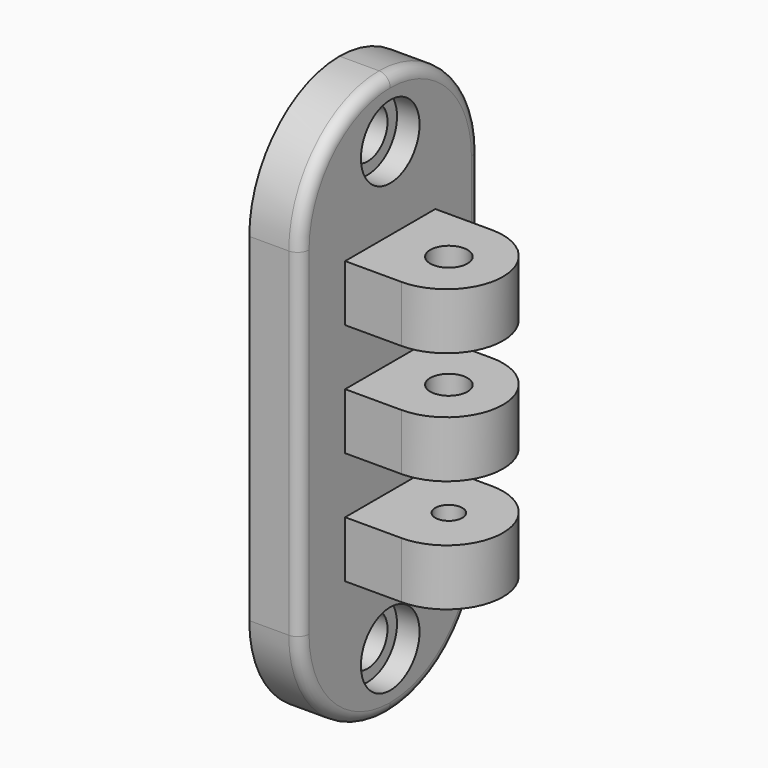
from build123d import *

# Parameters (mm, degrees)
F0_R          = 3.25
F0_W          = 10
F0_H          = 5
F0_R_2        = 2.2
F2_DEPTH      = 4.5
F3_DEPTH      = 10
F1_R          = 1.65
F1_R_2        = 1.2
F4_DEPTH      = 25
F5_DEPTH      = 2.5
F5_DEPTH_BACK = 12.5
F6_START      = -6.1
F6_DEPTH      = 8.5
F7_DEPTH      = 2
F8_R          = 1


with BuildPart() as f2:
    # F0 (on Right) → F2 (new body)
    with BuildSketch(Plane.YZ):
        with BuildLine():
            ThreePointArc((0, 25), (-7.0710678119, 22.0710678119), (-10, 15))
            Line((-10, 15), (-10, -15))
            ThreePointArc((-10, -15), (-7.0710678119, -22.0710678119), (0, -25))
            ThreePointArc((0, -25), (7.0710678119, -22.0710678119), (10, -15))
            Line((10, -15), (10, 15))
            ThreePointArc((10, 15), (7.0710678119, 22.0710678119), (0, 25))
        make_face()
        with Locations((0, -19.8)):
            Circle(F0_R, mode=Mode.SUBTRACT)
        with Locations((0, -10)):
            Rectangle(F0_W, F0_H, mode=Mode.SUBTRACT)
        Rectangle(F0_W, F0_H, mode=Mode.SUBTRACT)
        with Locations((0, 10)):
            Rectangle(F0_W, F0_H, mode=Mode.SUBTRACT)
        with Locations((0, 19.8)):
            Circle(F0_R, mode=Mode.SUBTRACT)
        with Locations((0, 10)):
            Rectangle(F0_W, F0_H)
        Rectangle(F0_W, F0_H)
        with Locations((0, -10)):
            Rectangle(F0_W, F0_H)
        with Locations((0, 19.8)):
            Circle(F0_R)
        with Locations((0, 19.8)):
            Circle(F0_R_2, mode=Mode.SUBTRACT)
        with Locations((0, -19.8)):
            Circle(F0_R)
        with Locations((0, -19.8)):
            Circle(F0_R_2, mode=Mode.SUBTRACT)
    extrude(amount=-F2_DEPTH)

    # F0 (on Right) → F3 (join)
    with BuildSketch(Plane.YZ):
        with Locations((0, 10)):
            Rectangle(F0_W, F0_H)
        Rectangle(F0_W, F0_H)
        with Locations((0, -10)):
            Rectangle(F0_W, F0_H)
    extrude(amount=F3_DEPTH)

    # F1 (on Top) → F4 (intersect, symmetric)
    with BuildSketch(Plane.XY):
        Polygon((0, -5), (0, 5), (0, 10), (-4.5, 10), (-4.5, -10), (0, -10), align=None)
        with BuildLine():
            Line((5, 5), (0, 5))
            Line((0, 5), (0, -5))
            Line((0, -5), (5, -5))
            ThreePointArc((5, -5), (8.5355339059, -3.5355339059), (10, 0))
            ThreePointArc((10, 0), (8.5355339059, 3.5355339059), (5, 5))
        make_face()
        with Locations((5.2, 0)):
            Circle(F1_R, mode=Mode.SUBTRACT)
        with Locations((5.2, 0)):
            Circle(F1_R)
        with Locations((5.2, 0)):
            Circle(F1_R_2, mode=Mode.SUBTRACT)
        with Locations((5.2, 0)):
            Circle(F1_R_2)
    extrude(amount=F4_DEPTH, both=True, mode=Mode.INTERSECT)

    # F1 (on Top) → F5 (cut, two sides)
    with BuildSketch(Plane.XY) as f5_sk:
        with Locations((5.2, 0)):
            Circle(F1_R)
        with Locations((5.2, 0)):
            Circle(F1_R_2, mode=Mode.SUBTRACT)
        with Locations((5.2, 0)):
            Circle(F1_R_2)
    extrude(amount=-F5_DEPTH, mode=Mode.SUBTRACT)
    extrude(f5_sk.sketch, amount=F5_DEPTH_BACK, mode=Mode.SUBTRACT)

    # F1 (on Top) → F6 (cut)
    with BuildSketch(Plane.XY.offset(F6_START)):
        with Locations((5.2, 0)):
            Circle(F1_R_2)
    extrude(amount=-F6_DEPTH, mode=Mode.SUBTRACT)

    # F0 (on Right) → F7 (cut)
    with BuildSketch(Plane.YZ):
        with Locations((0, 19.8)):
            Circle(F0_R)
        with Locations((0, 19.8)):
            Circle(F0_R_2, mode=Mode.SUBTRACT)
        with Locations((0, -19.8)):
            Circle(F0_R)
        with Locations((0, -19.8)):
            Circle(F0_R_2, mode=Mode.SUBTRACT)
    extrude(amount=-F7_DEPTH, mode=Mode.SUBTRACT)

    # F8
    f8_edges = [f2.edges().sort_by_distance(p)[0] for p in [
        (0, 10, 0),
        (0, 0, -25),
        (0, 0, 25),
        (0, -10, 0),
    ]]
    fillet(f8_edges, radius=F8_R)


solid = f2.part
